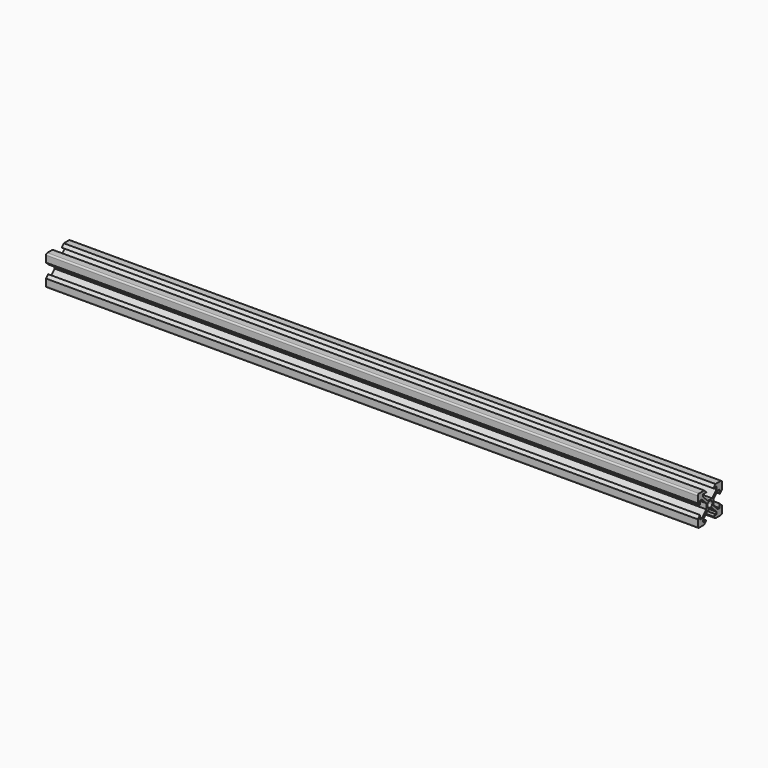
from build123d import *

# Parameters (mm, degrees)
F1_DEPTH = 431.8


# Not quite as in the source:
# - ends of sketch curves that miss each other by under 0.0002 mm in the source are joined


with BuildPart() as f1:
    # F0 (on Right) → F1 (new body)
    with BuildSketch(Plane.YZ):
        with BuildLine():
            Line((8.2, -10), (9, -10))
            ThreePointArc((9, -10), (9.7071067812, -9.7071067812), (10, -9))
            Line((10, -9), (10, -8.2))
            Line((10, -8.2), (8.2, -8.2))
            Line((8.2, -8.2), (8.2, -10))
        make_face()
        Polygon((5.4993398282, -8.2), (7.1393398282, -8.2), (5.4993398282, -6.56), align=None)
        Polygon((6.56, -5.4993398282), (8.2, -7.1393398282), (8.2, -5.4993398282), align=None)
        with BuildLine():
            Line((8.2, 10), (8.2, 8.2))
            Line((8.2, 8.2), (10, 8.2))
            Line((10, 8.2), (10, 9))
            ThreePointArc((10, 9), (9.7071067812, 9.7071067812), (9, 10))
            Line((9, 10), (8.2, 10))
        make_face()
        Polygon((8.2, 7.1393398282), (6.56, 5.4993398282), (8.2, 5.4993398282), align=None)
        Polygon((5.4993398282, 8.2), (5.4993398282, 6.56), (7.1393398282, 8.2), align=None)
        with BuildLine():
            Line((-9.9999004684, 8.2000055944), (-8.1999004684, 8.2000055944))
            Line((-8.1999004684, 8.2000055944), (-8.1999004684, 10.0000055944))
            Line((-8.1999004684, 10.0000055944), (-8.9999004684, 10.0000055944))
            ThreePointArc((-8.9999004684, 10.0000055944), (-9.7070072496, 9.7071123756), (-9.9999004684, 9.0000055944))
            Line((-9.9999004684, 9.0000055944), (-9.9999004684, 8.2000055944))
        make_face()
        Polygon((-7.1392402967, 8.2000055944), (-5.4992402967, 6.5600055944), (-5.4992402967, 8.2000055944), align=None)
        Polygon((-8.1999004684, 5.4993454226), (-6.5599004684, 5.4993454226), (-8.1999004684, 7.1393454226), align=None)
        with BuildLine():
            Line((-8.1999004684, -9.9999944056), (-8.1999004684, -8.1999944056))
            Line((-8.1999004684, -8.1999944056), (-9.9999004684, -8.1999944056))
            Line((-9.9999004684, -8.1999944056), (-9.9999004684, -8.9999944056))
            ThreePointArc((-9.9999004684, -8.9999944056), (-9.7070072496, -9.7071011868), (-8.9999004684, -9.9999944056))
            Line((-8.9999004684, -9.9999944056), (-8.1999004684, -9.9999944056))
        make_face()
        Polygon((-8.1999004684, -7.1393342338), (-6.5599004684, -5.4993342338), (-8.1999004684, -5.4993342338), align=None)
        Polygon((-5.4992402967, -8.1999944056), (-5.4992402967, -6.5599944056), (-7.1392402967, -8.1999944056), align=None)
        with BuildLine():
            Line((1.9173232366, -0.8566630648), (2.84, -1.7793398282))
            Line((2.84, -1.7793398282), (2.84, 0))
            Line((2.84, 0), (2.1, 0))
            ThreePointArc((2.1, 0), (2.0538231176, -0.4379618723), (1.9173232366, -0.8566630648))
        make_face()
        with BuildLine():
            Line((0, -2.84), (1.7793398282, -2.84))
            Line((1.7793398282, -2.84), (0.8566630648, -1.9173232366))
            ThreePointArc((0.8566630648, -1.9173232366), (0.4379618723, -2.0538231176), (0, -2.1))
            Line((0, -2.1), (0, -2.84))
        make_face()
        with BuildLine():
            Line((-1.7792402967, -2.8399944056), (9.95316e-05, -2.8399944056))
            Line((9.95316e-05, -2.8399944056), (0, -2.1))
            ThreePointArc((0, -2.1), (-0.4378623408, -2.0538175232), (-0.8565635332, -1.9173176422))
            Line((-0.8565635332, -1.9173176422), (-1.7792402967, -2.8399944056))
        make_face()
        Polygon((4.64, -10), (8.2, -10), (8.2, -8.2), (7.1393398282, -8.2), (5.4993398282, -8.2), (2.84, -8.2), align=None)
        Polygon((8.2, -8.2), (10, -8.2), (10, -4.64), (8.2, -2.84), (8.2, -5.4993398282), (8.2, -7.1393398282), align=None)
        with BuildLine():
            ThreePointArc((0, 2.1), (0.4379618723, 2.0538231176), (0.8566630648, 1.9173232366))
            Line((0.8566630648, 1.9173232366), (1.7793398282, 2.84))
            Line((1.7793398282, 2.84), (0, 2.84))
            Line((0, 2.84), (0, 2.1))
        make_face()
        with BuildLine():
            Line((2.1, 0), (2.84, 0))
            Line((2.84, 0), (2.84, 1.7793398282))
            Line((2.84, 1.7793398282), (1.9173232366, 0.8566630648))
            ThreePointArc((1.9173232366, 0.8566630648), (2.0538231176, 0.4379618723), (2.1, 0))
        make_face()
        with BuildLine():
            ThreePointArc((-0.8565635332, 1.917328831), (-0.4378623408, 2.053828712), (9.95316e-05, 2.1000055944))
            Line((9.95316e-05, 2.1000055944), (0, 2.84))
            Line((0, 2.84), (-1.7792402967, 2.8400055944))
            Line((-1.7792402967, 2.8400055944), (-0.8565635332, 1.917328831))
        make_face()
        Polygon((8.2, 8.2), (8.2, 7.1393398282), (8.2, 5.4993398282), (8.2, 2.84), (10, 4.64), (10, 8.2), align=None)
        Polygon((7.1393398282, 8.2), (8.2, 8.2), (8.2, 10), (4.64, 10), (2.84, 8.2), (5.4993398282, 8.2), align=None)
        with BuildLine():
            Line((-2.8399004684, 1.7793454226), (-2.8399004684, 5.5944e-06))
            Line((-2.8399004684, 5.5944e-06), (-2.0999004684, 5.5944e-06))
            ThreePointArc((-2.0999004684, 5.5944e-06), (-2.053723586, 0.4379674667), (-1.917223705, 0.8566686592))
            Line((-1.917223705, 0.8566686592), (-2.8399004684, 1.7793454226))
        make_face()
        Polygon((-8.1999004684, 10.0000055944), (-8.1999004684, 8.2000055944), (-7.1392402967, 8.2000055944), (-5.4992402967, 8.2000055944), (-2.8399004684, 8.2000055944), (-4.6399004684, 10.0000055944), align=None)
        Polygon((-8.1999004684, 5.4993454226), (-8.1999004684, 7.1393454226), (-8.1999004684, 8.2000055944), (-9.9999004684, 8.2000055944), (-9.9999004684, 4.6400055944), (-8.1999004684, 2.8400055944), align=None)
        with BuildLine():
            Line((-2.8399004684, 5.5944e-06), (-2.8399004684, -1.7793342338))
            Line((-2.8399004684, -1.7793342338), (-1.917223705, -0.8566574704))
            ThreePointArc((-1.917223705, -0.8566574704), (-2.053723586, -0.4379562779), (-2.0999004684, 5.5944e-06))
            Line((-2.0999004684, 5.5944e-06), (-2.8399004684, 5.5944e-06))
        make_face()
        Polygon((-9.9999004684, -8.1999944056), (-8.1999004684, -8.1999944056), (-8.1999004684, -7.1393342338), (-8.1999004684, -5.4993342338), (-8.1999004684, -2.8399944056), (-9.9999004684, -4.6399944056), align=None)
        Polygon((-5.4992402967, -8.1999944056), (-7.1392402967, -8.1999944056), (-8.1999004684, -8.1999944056), (-8.1999004684, -9.9999944056), (-4.6399004684, -9.9999944056), (-2.8399004684, -8.1999944056), align=None)
        with BuildLine():
            Line((-2.8399004684, -1.7793342338), (-1.7792402967, -2.8399944056))
            Line((-1.7792402967, -2.8399944056), (-0.8565635332, -1.9173176422))
            ThreePointArc((-0.8565635332, -1.9173176422), (-1.4848247089, -1.4849186461), (-1.917223705, -0.8566574704))
            Line((-1.917223705, -0.8566574704), (-2.8399004684, -1.7793342338))
        make_face()
        Polygon((-4.4695703825, -5.5303244915), (-1.7792402967, -2.8399944056), (-2.8399004684, -1.7793342338), (-5.5302305543, -4.4696643197), (-6.5599004684, -5.4993342338), (-8.1999004684, -7.1393342338), (-8.1999004684, -8.1999944056), (-7.1392402967, -8.1999944056), (-5.4992402967, -6.5599944056), align=None)
        with BuildLine():
            Line((7.1393398282, -8.2), (8.2, -8.2))
            Line((8.2, -8.2), (8.2, -7.1393398282))
            Line((8.2, -7.1393398282), (6.56, -5.4993398282))
            Line((6.56, -5.4993398282), (5.5303300859, -4.4696699141))
            Line((5.5303300859, -4.4696699141), (2.84, -1.7793398282))
            Line((2.84, -1.7793398282), (1.9173232366, -0.8566630648))
            ThreePointArc((1.9173232366, -0.8566630648), (1.4849242405, -1.4849242405), (0.8566630648, -1.9173232366))
            Line((0.8566630648, -1.9173232366), (1.7793398282, -2.84))
            Line((1.7793398282, -2.84), (4.4696699141, -5.5303300859))
            Line((4.4696699141, -5.5303300859), (5.4993398282, -6.56))
            Line((5.4993398282, -6.56), (7.1393398282, -8.2))
        make_face()
        with BuildLine():
            Line((1.9173232366, 0.8566630648), (2.84, 1.7793398282))
            Line((2.84, 1.7793398282), (5.5303300859, 4.4696699141))
            Line((5.5303300859, 4.4696699141), (6.56, 5.4993398282))
            Line((6.56, 5.4993398282), (8.2, 7.1393398282))
            Line((8.2, 7.1393398282), (8.2, 8.2))
            Line((8.2, 8.2), (7.1393398282, 8.2))
            Line((7.1393398282, 8.2), (5.4993398282, 6.56))
            Line((5.4993398282, 6.56), (4.4696699141, 5.5303300859))
            Line((4.4696699141, 5.5303300859), (1.7793398282, 2.84))
            Line((1.7793398282, 2.84), (0.8566630648, 1.9173232366))
            ThreePointArc((0.8566630648, 1.9173232366), (1.4849242405, 1.4849242405), (1.9173232366, 0.8566630648))
        make_face()
        with BuildLine():
            Line((-5.5302305543, 4.4696755085), (-2.8399004684, 1.7793454226))
            Line((-2.8399004684, 1.7793454226), (-1.917223705, 0.8566686592))
            ThreePointArc((-1.917223705, 0.8566686592), (-1.4848247089, 1.4849298349), (-0.8565635332, 1.917328831))
            Line((-0.8565635332, 1.917328831), (-1.7792402967, 2.8400055944))
            Line((-1.7792402967, 2.8400055944), (-4.4695703825, 5.5303356803))
            Line((-4.4695703825, 5.5303356803), (-5.4992402967, 6.5600055944))
            Line((-5.4992402967, 6.5600055944), (-7.1392402967, 8.2000055944))
            Line((-7.1392402967, 8.2000055944), (-8.1999004684, 8.2000055944))
            Line((-8.1999004684, 8.2000055944), (-8.1999004684, 7.1393454226))
            Line((-8.1999004684, 7.1393454226), (-6.5599004684, 5.4993454226))
            Line((-6.5599004684, 5.4993454226), (-5.5302305543, 4.4696755085))
        make_face()
    extrude(amount=F1_DEPTH)


solid = f1.part
